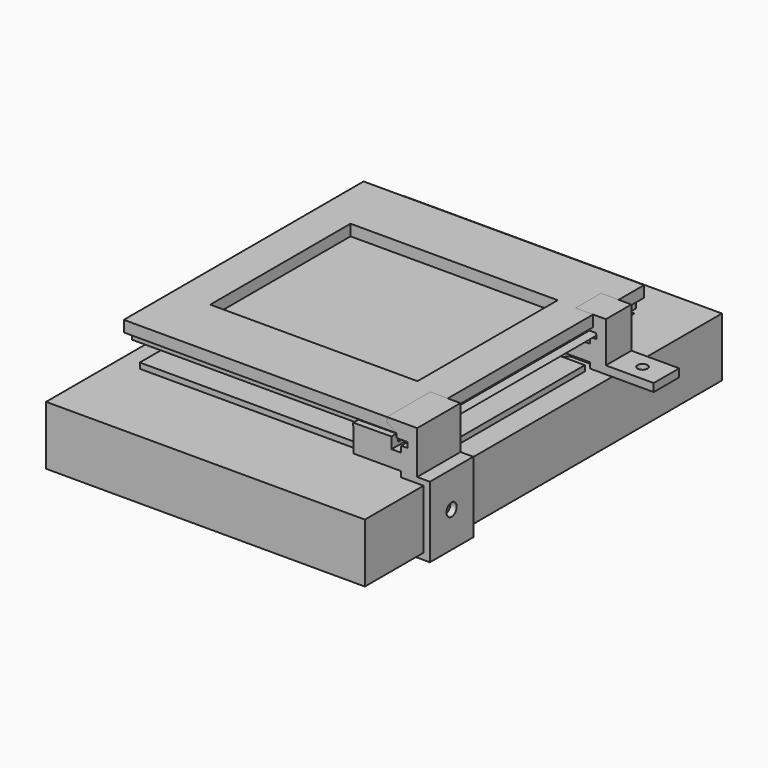
from build123d import *

# Parameters (mm, degrees)
F0_W           = 100
F0_H           = 140
F1_DEPTH       = 18.5
F3_DEPTH       = 1.75
F4_W           = 65
F4_H           = 55
F5_DEPTH       = 10
F6_W           = 88
F6_H           = 94
F6_W_2         = 86
F6_H_2         = 84
F6_W_3         = 65
F6_H_3         = 55
F6_H_4         = 3
F7_DEPTH       = 3.5
F8_DEPTH       = 2.5
F9_W           = 1
F9_H           = 1.25
F10_DEPTH      = 42
F10_DEPTH_BACK = 42
F12_DEPTH      = 47
F13_DEPTH      = 30
F15_DEPTH      = 12
F16_R          = 2
F17_DEPTH      = 3
F20_DEPTH      = 10
F21_R          = 1.55
F22_DEPTH      = 25


with BuildPart() as f1:
    # F0 (on Top) → F1 (new body)
    with BuildSketch(Plane.XY):
        Rectangle(F0_W, F0_H)
    extrude(amount=-F1_DEPTH)


with BuildPart() as f3:
    # F2 (on Top) → F3 (new body)
    with BuildSketch(Plane.XY):
        with BuildLine():
            Line((43, 42), (-43, 42))
            Line((-43, 42), (-43, 29))
            Line((-43, 29), (-36, 29))
            ThreePointArc((-36, 29), (-34, 27), (-36, 25))
            Line((-36, 25), (-43, 25))
            Line((-43, 25), (-43, -25))
            Line((-43, -25), (-36, -25))
            ThreePointArc((-36, -25), (-34, -27), (-36, -29))
            Line((-36, -29), (-43, -29))
            Line((-43, -29), (-43, -42))
            Line((-43, -42), (43, -42))
            Line((43, -42), (43, -29))
            Line((43, -29), (36, -29))
            ThreePointArc((36, -29), (34, -27), (36, -25))
            Line((36, -25), (43, -25))
            Line((43, -25), (43, 25))
            Line((43, 25), (36, 25))
            ThreePointArc((36, 25), (34, 27), (36, 29))
            Line((36, 29), (43, 29))
            Line((43, 29), (43, 42))
        make_face()
    extrude(amount=F3_DEPTH)


with BuildPart() as f5:
    # F4 (on face) → F5 (new body)
    with BuildSketch(Plane.XY.offset(1.75)):
        Rectangle(F4_W, F4_H)
    extrude(amount=F5_DEPTH)


with BuildPart() as f7:
    # F6 (on face) → F7 (new body)
    with BuildSketch(Plane.XY.offset(11.75)):
        Rectangle(F6_W, F6_H)
        Polygon((-43, 42), (-43, 45), (43, 45), (43, 42), (43, -42), (43, -44), (43, -45), (-43, -45), (-43, -44), (-43, -42), align=None, mode=Mode.SUBTRACT)
        Rectangle(F6_W_2, F6_H_2)
        Rectangle(F6_W_3, F6_H_3, mode=Mode.SUBTRACT)
        with Locations((0, 43.5)):
            Rectangle(F6_W_2, F6_H_4)
        Polygon((43, -42), (-43, -42), (-43, -44), (-43, -45), (43, -45), (43, -44), align=None)
    extrude(amount=F7_DEPTH)

    # F6 (on face) → F8 (join)
    with BuildSketch(Plane.XY.offset(11.75)):
        with Locations((0, 43.5)):
            Rectangle(F6_W_2, F6_H_4)
        Polygon((43, -42), (-43, -42), (-43, -44), (-43, -45), (43, -45), (43, -44), align=None)
    extrude(amount=-F8_DEPTH)

    # F9 (on Front) → F10 (join, two sides)
    with BuildSketch(Plane.XZ) as f10_sk:
        with Locations((42.5, 9.125)):
            Rectangle(F9_W, F9_H)
        Polygon((43, 9.75), (43, 8.5), (45, 9.75), align=None)
    extrude(amount=F10_DEPTH)
    extrude(f10_sk.sketch, amount=-F10_DEPTH_BACK)


with BuildPart() as f12:
    # F11 (on Front) → F12 (new body)
    with BuildSketch(Plane.XZ):
        Polygon((27.9699712028, 6.7499098263), (28, 1.75), (43, 1.75), (43, 0), (48, 0), (50, 0), (52, 0), (52, 1.75), (48, 1.75), (48, 13.75), (48, 15.25), (38.5, 15.25), (38.5, 13.75), (41.5, 11.875), (41.5, 10.4472711682), (44.9731051922, 10.4472711682), (45, 8.7854899466), (43, 8.7531212961), (43, 6.8401781918), align=None)
        Polygon((52, 0), (50, 0), (50, -18.5), (35.7036739588, -18.5), (35.7036739588, -20.5), (52, -20.5), align=None)
    extrude(amount=F12_DEPTH)

    # F11 (on Front) → F13 (cut)
    with BuildSketch(Plane.XZ):
        Polygon((27.9699712028, 6.7499098263), (28, 1.75), (43, 1.75), (43, 0), (48, 0), (50, 0), (52, 0), (52, 1.75), (48, 1.75), (48, 13.75), (48, 15.25), (38.5, 15.25), (38.5, 13.75), (41.5, 11.875), (41.5, 10.4472711682), (44.9731051922, 10.4472711682), (45, 8.7854899466), (43, 8.7531212961), (43, 6.8401781918), align=None)
        Polygon((52, 0), (50, 0), (50, -18.5), (35.7036739588, -18.5), (35.7036739588, -20.5), (52, -20.5), align=None)
    extrude(amount=F13_DEPTH, mode=Mode.SUBTRACT)

    # F14 (on face) → F15 (join)
    with BuildSketch(Plane(origin=(28.0094999534, 0, 0.1682213529), x_dir=(0, -1, 0), z_dir=(-0.9999819653, 0, -0.0060057594))):
        Polygon((39.5, 5.9370710514), (47, 5.9370710514), (47, 7.0816674463), (47, 10.0810629427), (44.5, 10.0810629427), (44.5, 7.5816674463), (42, 7.5816674463), (42, 9.5810629427), (42, 10.0810629427), (39.5, 10.0810629427), (39.5, 9.5810629427), align=None)
    extrude(amount=-F15_DEPTH)

    # F16 (on face) → F17 (cut)
    with BuildSketch(Plane.YZ.offset(52)):
        with Locations((-38.5, -9.375)):
            Circle(F16_R)
    extrude(amount=-F17_DEPTH, mode=Mode.SUBTRACT)


with BuildPart() as f20:
    # F19 (on offset) → F20 (new body)
    with BuildSketch(Plane(origin=(0, 27, 0), x_dir=(-1, 0, 0), z_dir=(0, 1, 0))):
        Polygon((-43, 1.75), (-28, 1.75), (-27.9699712028, 6.7499098263), (-43, 6.8401781918), (-43, 8.7531212961), (-45, 8.7854899466), (-44.9731051922, 10.4472711682), (-41.5, 10.4472711682), (-41.5, 11.875), (-38.5, 13.75), (-38.5, 15.25), (-48, 15.25), (-48, 2.5), (-63, 2.5), (-63, 0), (-43, 0), align=None)
    extrude(amount=F20_DEPTH)

    # F21 (on face) → F22 (cut)
    with BuildSketch(Plane.XY.offset(2.5)):
        with Locations((55.5, 32)):
            Circle(F21_R)
    extrude(amount=-F22_DEPTH, mode=Mode.SUBTRACT)


solid = Compound([f1.part, f3.part, f5.part, f7.part, f12.part, f20.part])
